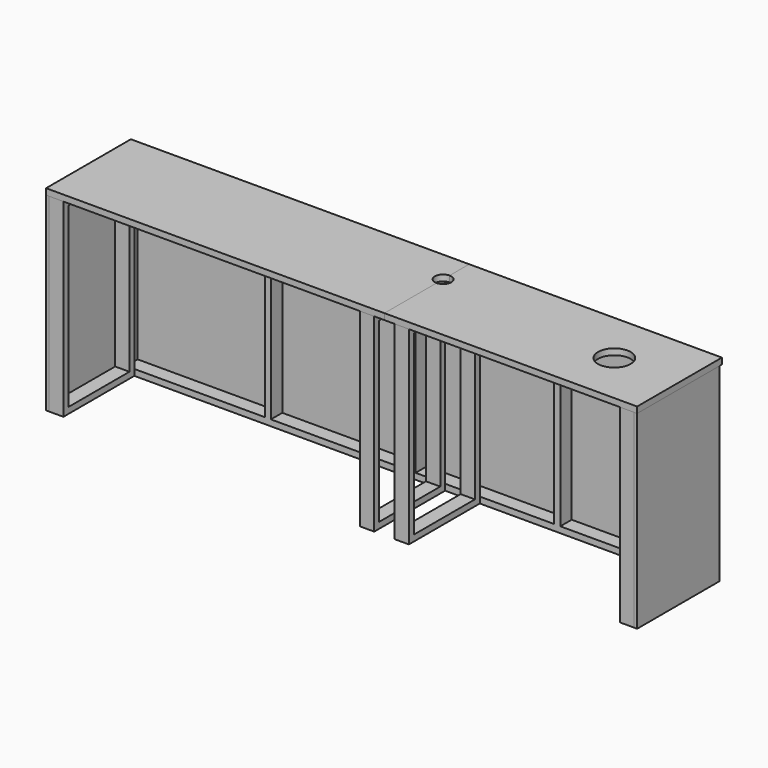
from build123d import *

# Parameters (mm, degrees)
F0_W      = 3644.9
F0_H      = 1181.1
F0_W_2    = 38.1
F0_H_2    = 1104.9
F1_DEPTH  = 88.9
F2_W      = 3644.9
F2_H      = 1181.1
F3_DEPTH  = 19.05
F4_W      = 2089.15
F4_H      = 19.05
F5_DEPTH  = 38.1
F4_R      = 101.6
F4_W_2    = 1555.75
F6_DEPTH  = 38.1
F7_W      = 552.45
F7_H      = 1181.1
F7_W_2    = 476.25
F7_H_2    = 1104.9
F8_DEPTH  = 88.9
F9_W      = 552.45
F9_H      = 1181.1
F9_W_2    = 476.25
F9_H_2    = 1104.9
F10_DEPTH = 88.9
F11_W     = 641.35
F11_H     = 1181.1
F12_DEPTH = 19.05
F13_W     = 19.05
F13_H     = 1181.1
F13_W_2   = 641.35
F14_DEPTH = 19.05
F15_W     = 88.9
F15_H     = 1104.9
F15_H_2   = 38.1
F16_DEPTH = 552.45
F17_W     = 476.25
F17_H     = 1104.9
F18_DEPTH = 88.9
F19_W     = 88.9
F19_H     = 1104.9
F19_H_2   = 38.1
F20_DEPTH = 552.45
F21_W     = 476.25
F21_H     = 1104.9
F22_DEPTH = 88.9


# Not quite as in the source:
# - a feature names something its author has since deleted; it is built from what else it names


with BuildPart() as f1:
    # F0 (on Front) → F1 (new body)
    with BuildSketch(Plane.XZ):
        with Locations((1822.45, 590.55)):
            Rectangle(F0_W, F0_H)
        Polygon((38.1, 38.1), (38.1, 1143), (901.7, 1143), (939.8, 1143), (1803.4, 1143), (1841.5, 1143), (2705.1, 1143), (2743.2, 1143), (3606.8, 1143), (3606.8, 38.1), (2743.2, 38.1), (2705.1, 38.1), (1841.5, 38.1), (1803.4, 38.1), (939.8, 38.1), (901.7, 38.1), align=None, mode=Mode.SUBTRACT)
        with Locations((920.75, 590.55)):
            Rectangle(F0_W_2, F0_H_2)
        with Locations((1822.45, 590.55)):
            Rectangle(F0_W_2, F0_H_2)
        with Locations((2724.15, 590.55)):
            Rectangle(F0_W_2, F0_H_2)
    extrude(amount=F1_DEPTH)


with BuildPart() as f3:
    # F2 (on face) → F3 (new body)
    with BuildSketch(Plane(origin=(0, 0, 0), x_dir=(-1, 0, 0), z_dir=(0, 1, 0))):
        with Locations((-1822.45, 590.55)):
            Rectangle(F2_W, F2_H)
    extrude(amount=F3_DEPTH)


with BuildPart() as f5:
    # F4 (on face) → F5 (new body)
    with BuildSketch(Plane.XY.offset(1181.1)):
        with Locations((1044.575, 9.525)):
            Rectangle(F4_W, F4_H)
        with BuildLine():
            ThreePointArc((2089.15, -234.95), (2038.35, -184.15), (2089.15, -133.35))
            Line((2089.15, -133.35), (2089.15, 0))
            Line((2089.15, 0), (0, 0))
            Line((0, 0), (0, 19.05))
            Line((0, 19.05), (-19.05, 19.05))
            Line((-19.05, 19.05), (-19.05, -641.35))
            Line((-19.05, -641.35), (2089.15, -641.35))
            Line((2089.15, -641.35), (2089.15, -234.95))
        make_face()
    extrude(amount=F5_DEPTH)


with BuildPart() as f6:
    # F4 (on face) → F6 (new body)
    with BuildSketch(Plane.XY.offset(1181.1)):
        with BuildLine():
            ThreePointArc((2089.15, -133.35), (2125.0710244843, -148.2289755157), (2139.95, -184.15))
            ThreePointArc((2139.95, -184.15), (2125.0710244843, -220.0710244843), (2089.15, -234.95))
            Line((2089.15, -234.95), (2089.15, -641.35))
            Line((2089.15, -641.35), (3663.95, -641.35))
            Line((3663.95, -641.35), (3663.95, 19.05))
            Line((3663.95, 19.05), (3644.9, 19.05))
            Line((3644.9, 19.05), (3644.9, 0))
            Line((3644.9, 0), (2089.15, 0))
            Line((2089.15, 0), (2089.15, -133.35))
        make_face()
        with Locations((3257.55, -311.15)):
            Circle(F4_R, mode=Mode.SUBTRACT)
        with Locations((2867.025, 9.525)):
            Rectangle(F4_W_2, F4_H)
    extrude(amount=F6_DEPTH)


with BuildPart() as f8:
    # F7 (on face) → F8 (new body)
    with BuildSketch(Plane(origin=(0, 0, 0), x_dir=(0, -1, 0), z_dir=(-1, 0, 0))):
        with Locations((365.125, 590.55)):
            Rectangle(F7_W, F7_H)
        with Locations((365.125, 590.55)):
            Rectangle(F7_W_2, F7_H_2, mode=Mode.SUBTRACT)
    extrude(amount=-F8_DEPTH)


with BuildPart() as f10:
    # F9 (on face) → F10 (new body)
    with BuildSketch(Plane.YZ.offset(3644.9)):
        with Locations((-365.125, 590.55)):
            Rectangle(F9_W, F9_H)
        with Locations((-365.125, 590.55)):
            Rectangle(F9_W_2, F9_H_2, mode=Mode.SUBTRACT)
    extrude(amount=-F10_DEPTH)


with BuildPart() as f12:
    # F11 (on face) → F12 (new body)
    with BuildSketch(Plane.YZ.offset(3644.9)):
        with Locations((-320.675, 590.55)):
            Rectangle(F11_W, F11_H)
    extrude(amount=F12_DEPTH)


with BuildPart() as f14:
    # F13 (on face) → F14 (new body)
    with BuildSketch(Plane(origin=(0, 0, 0), x_dir=(0, -1, 0), z_dir=(-1, 0, 0))):
        with Locations((-9.525, 590.55)):
            Rectangle(F13_W, F13_H)
        with Locations((320.675, 590.55)):
            Rectangle(F13_W_2, F13_H)
    extrude(amount=F14_DEPTH)


with BuildPart() as f16:
    # F15 (on face) → F16 (new body)
    with BuildSketch(Plane.XZ.offset(88.9)):
        Polygon((2152.65, 1181.1), (2152.65, 1143), (2241.55, 1143), (2241.55, 1181.1), (2216.15, 1181.1), align=None)
        with Locations((2197.1, 590.55)):
            Rectangle(F15_W, F15_H)
        with Locations((2197.1, 19.05)):
            Rectangle(F15_W, F15_H_2)
    extrude(amount=F16_DEPTH)

    # F17 (on face) → F18 (cut, through all)
    with BuildSketch(Plane.YZ.offset(2241.55)):
        with Locations((-365.125, 590.55)):
            Rectangle(F17_W, F17_H)
    extrude(amount=-F18_DEPTH, mode=Mode.SUBTRACT)


with BuildPart() as f20:
    # F19 (on face) → F20 (new body)
    with BuildSketch(Plane.XZ.offset(88.9)):
        with Locations((1981.2, 590.55)):
            Rectangle(F19_W, F19_H)
        with Locations((1981.2, 1162.05)):
            Rectangle(F19_W, F19_H_2)
        with Locations((1981.2, 19.05)):
            Rectangle(F19_W, F19_H_2)
    extrude(amount=F20_DEPTH)

    # F21 (on face) → F22 (cut, through all)
    with BuildSketch(Plane(origin=(1936.75, 0, 0), x_dir=(0, -1, 0), z_dir=(-1, 0, 0))):
        with Locations((365.125, 590.55)):
            Rectangle(F21_W, F21_H)
    extrude(amount=-F22_DEPTH, mode=Mode.SUBTRACT)


solid = Compound([f1.part, f3.part, f5.part, f6.part, f8.part, f10.part, f12.part, f14.part, f16.part, f20.part])
